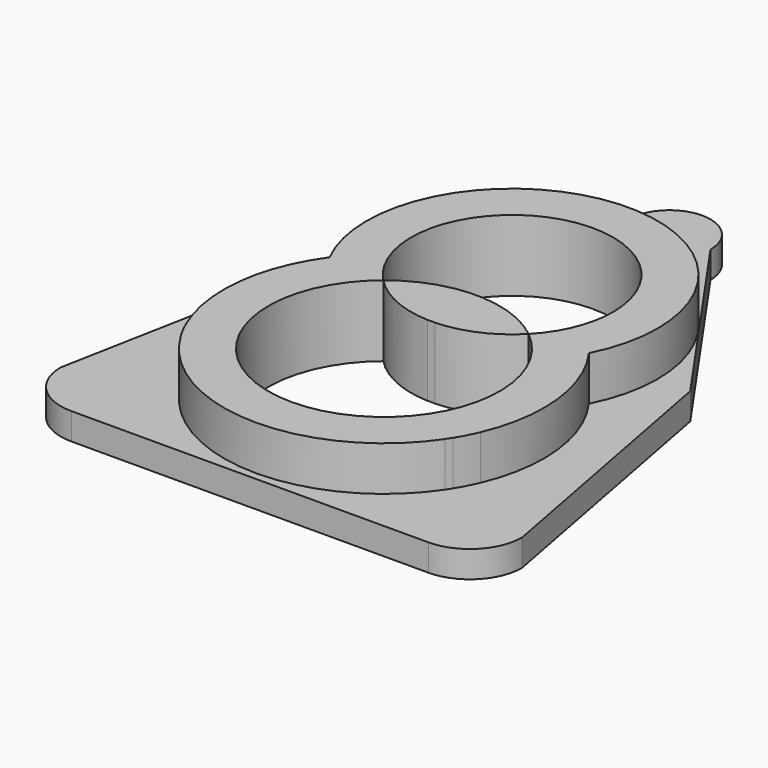
from build123d import *

# Parameters (mm, degrees)
F1_DEPTH = 203.2
F2_DEPTH = 76.2
F3_DEPTH = 76.2


with BuildPart() as f1:
    # F0 (on Top) → F1 (new body)
    with BuildSketch(Plane.XY):
        with BuildLine():
            ThreePointArc((419.7935890943, -179.8970573523), (447.3902688574, -91.8235047271), (456.7161138921, 0))
            ThreePointArc((456.7161138921, 0), (434.4385486274, 140.8998089254), (369.7791499823, 268.054078363))
            ThreePointArc((369.7791499823, 268.054078363), (325.2928462726, 320.5841119777), (273.4170123321, 365.8315815455))
            ThreePointArc((273.4170123321, 365.8315815455), (246.4421811438, 307.4408238889), (207.1859726201, 256.489158659))
            ThreePointArc((207.1859726201, 256.489158659), (297.5107304832, 142.1269890184), (329.7161138921, 0))
            ThreePointArc((329.7161138921, 0), (-142.1269890184, -297.5107304832), (-207.1859726201, 256.489158659))
            ThreePointArc((-207.1859726201, 256.489158659), (-246.4421811438, 307.4408238889), (-273.4170123321, 365.8315815455))
            ThreePointArc((-273.4170123321, 365.8315815455), (-325.2928462726, 320.5841119777), (-369.7791499823, 268.054078363))
            ThreePointArc((-369.7791499823, 268.054078363), (-453.8864585085, 50.7611216519), (-419.8593220682, -179.7435905981))
            ThreePointArc((-419.8593220682, -179.7435905981), (-406.5468550807, -208.1087775964), (-391.3208220922, -235.4944221967))
            ThreePointArc((-391.3208220922, -235.4944221967), (-382.2017695395, -248.0670908962), (-374.4319310628, -261.5154635758))
            ThreePointArc((-374.4319310628, -261.5154635758), (3.5288735732, -456.7024805494), (378.4283659046, -255.6982216744))
            ThreePointArc((378.4283659046, -255.6982216744), (383.1851939749, -247.8182784421), (388.4206166967, -240.2478578752))
            ThreePointArc((388.4206166967, -240.2478578752), (405.232162336, -210.6573124702), (419.7935890943, -179.8970573523))
        make_face()
        with BuildLine():
            ThreePointArc((273.4170123321, 365.8315815455), (325.2928462726, 320.5841119777), (369.7791499823, 268.054078363))
            ThreePointArc((369.7791499823, 268.054078363), (385.986239752, 609.5055315027), (140.4677009498, 847.3550883961))
            ThreePointArc((140.4677009498, 847.3550883961), (1.9062997603, 871.8382036836), (-136.8741128131, 848.6286815054))
            ThreePointArc((-136.8741128131, 848.6286815054), (-385.2805466524, 611.2764056323), (-369.7791499823, 268.054078363))
            ThreePointArc((-369.7791499823, 268.054078363), (-325.2928462726, 320.5841119777), (-273.4170123321, 365.8315815455))
            ThreePointArc((-273.4170123321, 365.8315815455), (-46.0335917284, 741.1414455435), (288.1264667684, 456.7161138921))
            ThreePointArc((288.1264667684, 456.7161138921), (284.4253316514, 410.6825221637), (273.4170123321, 365.8315815455))
        make_face()
    extrude(amount=F1_DEPTH)

    # F0 (on Top) → F2 (join)
    with BuildSketch(Plane.XY):
        with BuildLine():
            ThreePointArc((-136.8741128131, 848.6286815054), (1.9062997603, 871.8382036836), (140.4677009498, 847.3550883961))
            Line((140.4677009498, 847.3550883961), (116.8562267222, 1017.7334547043))
            ThreePointArc((116.8562267222, 1017.7334547043), (-6.6232636312, 901.0650780865), (-116.1054302545, 1030.9586877525))
            Line((-116.1054302545, 1030.9586877525), (-136.8741128131, 848.6286815054))
        make_face()
        with BuildLine():
            ThreePointArc((-369.7791499823, 268.054078363), (-385.2805466524, 611.2764056323), (-136.8741128131, 848.6286815054))
            Line((-136.8741128131, 848.6286815054), (-116.1054302545, 1030.9586877525))
            Line((-116.1054302545, 1030.9586877525), (-508, 456.7161138921))
            Line((-508, 456.7161138921), (-647.4473526625, -274.5237812852))
            ThreePointArc((-647.4473526625, -274.5237812852), (-592.3042832709, -205.6816607537), (-508, -179.7435905981))
            Line((-508, -179.7435905981), (-419.8593220682, -179.7435905981))
            ThreePointArc((-419.8593220682, -179.7435905981), (-453.8864585085, 50.7611216519), (-369.7791499823, 268.054078363))
        make_face()
        with BuildLine():
            ThreePointArc((369.7791499823, 268.054078363), (434.4385486274, 140.8998089254), (456.7161138921, 0))
            ThreePointArc((456.7161138921, 0), (447.3902688574, -91.8235047271), (419.7935890943, -179.8970573523))
            Line((419.7935890943, -179.8970573523), (508, -179.8970573523))
            ThreePointArc((508, -179.8970573523), (591.7238414708, -205.718805945), (646.3592496941, -274.212721728))
            Line((646.3592496941, -274.212721728), (508, 456.7161138919))
            Line((508, 456.7161138919), (116.8562267222, 1017.7334547043))
            Line((116.8562267222, 1017.7334547043), (140.4677009498, 847.3550883961))
            ThreePointArc((140.4677009498, 847.3550883961), (385.986239752, 609.5055315027), (369.7791499823, 268.054078363))
        make_face()
        with BuildLine():
            Line((508, -179.8970573523), (419.7935890943, -179.8970573523))
            ThreePointArc((419.7935890943, -179.8970573523), (405.232162336, -210.6573124702), (388.4206166967, -240.2478578752))
            ThreePointArc((388.4206166967, -240.2478578752), (441.0271546914, -195.8397204001), (508, -179.8970573523))
        make_face()
        with BuildLine():
            ThreePointArc((508, -477.1830565354), (379.6992396403, -403.597742884), (378.4283659046, -255.6982216744))
            ThreePointArc((378.4283659046, -255.6982216744), (3.5288735732, -456.7024805494), (-374.4319310628, -261.5154635758))
            ThreePointArc((-374.4319310628, -261.5154635758), (-362.1862522373, -294.6432083013), (-358.027476706, -329.7161138921))
            ThreePointArc((-358.027476706, -329.7161138921), (-401.8227065948, -435.6318356161), (-507.6300820622, -479.6881809709))
            Line((-507.6300820622, -479.6881809709), (508, -477.1830565354))
        make_face()
        with BuildLine():
            ThreePointArc((-391.3208220922, -235.4944221967), (-406.5468550807, -208.1087775964), (-419.8593220682, -179.7435905981))
            Line((-419.8593220682, -179.7435905981), (-508, -179.7435905981))
            ThreePointArc((-508, -179.7435905981), (-443.3428546463, -194.3971895028), (-391.3208220922, -235.4944221967))
        make_face()
    extrude(amount=F2_DEPTH)

    # F0 (on Top) → F3 (join)
    with BuildSketch(Plane.XY):
        with BuildLine():
            ThreePointArc((508, -179.8970573523), (441.0271546914, -195.8397204001), (388.4206166967, -240.2478578752))
            ThreePointArc((388.4206166967, -240.2478578752), (383.5023063354, -248.0233652786), (378.4283659046, -255.6982216744))
            ThreePointArc((378.4283659046, -255.6982216744), (379.6992396403, -403.597742884), (508, -477.1830565354))
            ThreePointArc((508, -477.1830565354), (613.1064729871, -433.646529931), (656.6429995915, -328.5400569439))
            Line((656.6429995915, -328.5400569439), (646.3592496941, -274.212721728))
            ThreePointArc((646.3592496941, -274.212721728), (591.7238414708, -205.718805945), (508, -179.8970573523))
        make_face()
        with BuildLine():
            ThreePointArc((-358.027476706, -329.7161138921), (-362.1862522373, -294.6432083013), (-374.4319310628, -261.5154635758))
            ThreePointArc((-374.4319310628, -261.5154635758), (-383.0973680277, -248.6483768275), (-391.3208220922, -235.4944221967))
            ThreePointArc((-391.3208220922, -235.4944221967), (-443.3428546463, -194.3971895028), (-508, -179.7435905981))
            ThreePointArc((-508, -179.7435905981), (-592.3042832709, -205.6816607537), (-647.4473526625, -274.5237812852))
            Line((-647.4473526625, -274.5237812852), (-657.972523294, -329.7161138921))
            ThreePointArc((-657.972523294, -329.7161138921), (-613.915721724, -435.8934072973), (-507.6300820622, -479.6881809709))
            ThreePointArc((-507.6300820622, -479.6881809709), (-401.8227065948, -435.6318356161), (-358.027476706, -329.7161138921))
        make_face()
        with BuildLine():
            ThreePointArc((-116.1054302545, 1030.9586877525), (-6.6232636312, 901.0650780865), (116.8562267222, 1017.7334547043))
            ThreePointArc((116.8562267222, 1017.7334547043), (6.6232636312, 1134.401831322), (-116.1054302545, 1030.9586877525))
        make_face()
    extrude(amount=F3_DEPTH)


with BuildPart() as f1b:
    # F0 (on Top) → F1, piece 2 (new body)
    with BuildSketch(Plane.XY):
        with BuildLine():
            ThreePointArc((10.9918600793, 168.7993900561), (117.5702579301, 193.6684085178), (207.1859726201, 256.489158659))
            ThreePointArc((207.1859726201, 256.489158659), (0, 329.7161138921), (-207.1859726201, 256.489158659))
            ThreePointArc((-207.1859726201, 256.489158659), (-117.5702579301, 193.6684085178), (-10.9918600793, 168.7993900561))
            ThreePointArc((-10.9918600793, 168.7993900561), (0, 169.1568948383), (10.9918600793, 168.7993900561))
        make_face()
    extrude(amount=F1_DEPTH)


solid = Compound([f1.part, f1b.part])
